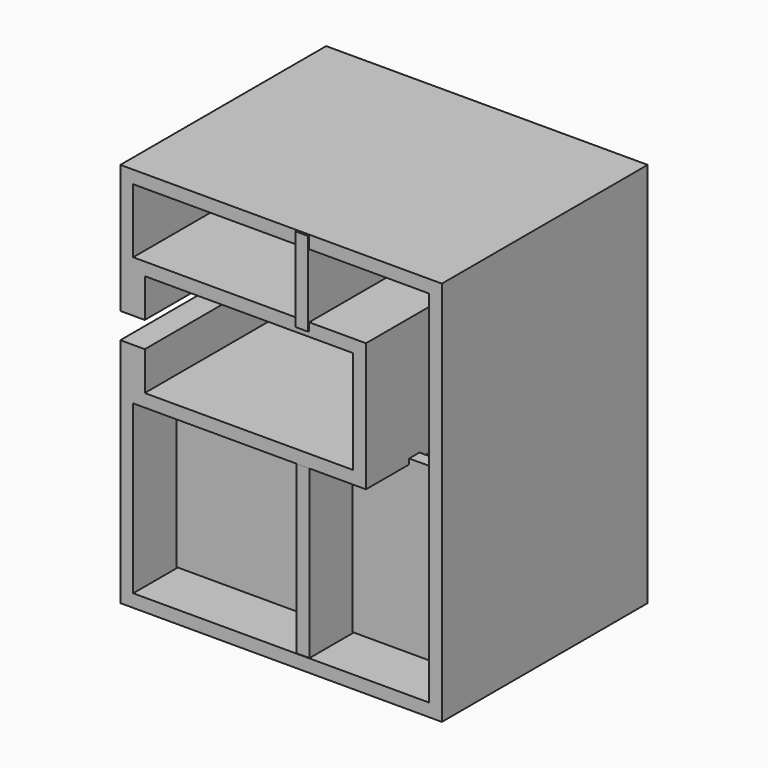
from build123d import *

# Parameters (mm, degrees)
F0_W         = 63.5
F0_H         = 50.8
F1_DEPTH     = 76.2
F3_DEPTH     = 38.1
F4_T         = 2.54
F4_T3_DEPTH  = 9.906
F4_T5_DEPTH  = 46.228
F4_T7_DEPTH  = 12.7
F4_T9_DEPTH  = 12.7
F4_T11_DEPTH = 25.4
F4_T13_DEPTH = 43.18
F5_W         = 49.4960099459
F5_H         = 36.6942100227
F5_W_2       = 49.6212309226
F5_H_2       = 16.634516418
F6_DEPTH     = 1.27
F7_W         = 57.8342098743
F7_H         = 36.6147905588
F8_DEPTH     = 1.27
F10_W        = 61.5059640259
F10_H        = 33.8196810335
F11_DEPTH    = 1.27


# Not quite as in the source:
# - a shell that OpenCascade refuses in one call is made with other operations: the cavity is built on its own and cut out


with BuildPart() as f1:
    # F0 (on Top) → F1 (new body)
    with BuildSketch(Plane.XY):
        with Locations((-4.2696721688, -14.4747652373)):
            Rectangle(F0_W, F0_H)
    extrude(amount=F1_DEPTH)

    # F2 (on face) → F3 (cut)
    with BuildSketch(Plane.XZ.offset(39.8747652373)):
        Polygon((9.9543278312, 58.42), (-31.1936721688, 58.42), (-31.1936721688, 50.8), (-39.8653410375, 50.8), (-39.8653410375, 45.72), (-31.1936721688, 45.72), (-31.1936721688, 38.1), (9.9543278312, 38.1), align=None)
    extrude(amount=-F3_DEPTH, mode=Mode.SUBTRACT)

    # F4: shell of thickness 2.54, made by hand


with BuildPart() as f4_core1:
    # F4_t2: copy of F1
    add(f1.part)

    # the walls: a layer under each face that stays
    f4_faces = [f4_core1.faces().sort_by_distance(p)[0] for p in [
        (-4.2696721688, 10.9252347627, 38.1),
        (27.4803278312, -14.4747652373, 38.1),
        (-36.0196721688, -14.4747652373, 38.1),
        (-4.2696721688, -14.4747652373, 0),
        (-4.2696721688, -14.4747652373, 76.2),
        (-33.6066721688, -20.8247652373, 45.72),
        (-13.0326721688, -1.7747652373, 48.26),
        (-33.6066721688, -20.8247652373, 50.8),
        (-31.1936721688, -20.8247652373, 54.61),
        (-10.6196721688, -20.8247652373, 58.42),
        (9.9543278312, -20.8247652373, 48.26),
        (-10.6196721688, -20.8247652373, 38.1),
        (-31.1936721688, -20.8247652373, 41.91),
    ]]
    thicken(f4_faces, amount=-F4_T, mode=Mode.SUBTRACT)

    # F4_s4 → F4_t3 (cut)
    with BuildSketch(Plane.YZ.offset(-38.5596721688)):
        Polygon((-1.8001652373, 45.7454), (-1.7747652373, 43.18), (0.7652347627, 43.18), (0.7652347627, 45.72), align=None)
        Polygon((-1.8001652373, 50.7746), (0.7652347627, 50.8), (0.7652347627, 53.34), (-1.7747652373, 53.34), align=None)
    extrude(amount=F4_T3_DEPTH, mode=Mode.SUBTRACT)

    # F4_s6 → F4_t5 (cut)
    with BuildSketch(Plane.YZ.offset(-33.7336721688)):
        Polygon((-1.8001652373, 38.1254), (0.7652347627, 38.1), (0.7652347627, 35.56), (-1.7747652373, 35.56), align=None)
        Polygon((-1.8001652373, 58.3946), (0.7652347627, 58.42), (0.7652347627, 60.96), (-1.7747652373, 60.96), align=None)
    extrude(amount=F4_T5_DEPTH, mode=Mode.SUBTRACT)

    # F4_s8 → F4_t7 (cut)
    with BuildSketch(Plane.XY.offset(35.56)):
        Polygon((-31.1682721688, -1.8001652373), (-31.1936721688, 0.7652347627), (-33.7336721688, 0.7652347627), (-33.7336721688, -1.7747652373), align=None)
    extrude(amount=F4_T7_DEPTH, mode=Mode.SUBTRACT)

    # F4_s10 → F4_t9 (cut)
    with BuildSketch(Plane.XY.offset(48.26)):
        Polygon((-31.1682721688, -1.8001652373), (-31.1936721688, 0.7652347627), (-33.7336721688, 0.7652347627), (-33.7336721688, -1.7747652373), align=None)
    extrude(amount=F4_T9_DEPTH, mode=Mode.SUBTRACT)

    # F4_s12 → F4_t11 (cut)
    with BuildSketch(Plane.XY.offset(35.56)):
        Polygon((9.9289278312, -1.8001652373), (9.9543278312, 0.7652347627), (12.4943278312, 0.7652347627), (12.4943278312, -1.7747652373), align=None)
    extrude(amount=F4_T11_DEPTH, mode=Mode.SUBTRACT)

    # F4_s14 → F4_t13 (cut)
    with BuildSketch(Plane.XZ.offset(-0.7652347627)):
        Polygon((-31.1682721688, 58.3946), (-33.7336721688, 58.42), (-33.7336721688, 60.96), (-31.1936721688, 60.96), align=None)
        Polygon((9.9289278312, 58.3946), (9.9543278312, 60.96), (12.4943278312, 60.96), (12.4943278312, 58.42), align=None)
        Polygon((9.9289278312, 38.1254), (12.4943278312, 38.1), (12.4943278312, 35.56), (9.9543278312, 35.56), align=None)
        Polygon((-31.1682721688, 38.1254), (-31.1936721688, 35.56), (-33.7336721688, 35.56), (-33.7336721688, 38.1), align=None)
    extrude(amount=F4_T13_DEPTH, mode=Mode.SUBTRACT)


with BuildPart() as f1_1:
    add(f1.part)

    # what is left inside the walls is the cavity
    f4_cavity = [f4_core1.part.solids().sort_by_distance(p)[0] for p in [
        (-4.269672, 8.359835, 49.953333),
    ]]
    add(f4_cavity, mode=Mode.SUBTRACT)

    # F5 (on Right) → F6 (join, symmetric)
    with BuildSketch(Plane.YZ):
        with Locations((-15.0325410068, 18.3471050113)):
            Rectangle(F5_W, F5_H)
        with Locations((-15.3072369285, 67.7350275218)):
            Rectangle(F5_W_2, F5_H_2)
    extrude(amount=F6_DEPTH, both=True)

    # F7 (on Front) → F8 (join, symmetric)
    with BuildSketch(Plane.XZ):
        with Locations((-4.0594032034, 18.3073952794)):
            Rectangle(F7_W, F7_H)
    extrude(amount=F8_DEPTH, both=True)

    # F10 (on offset) → F11 (join, symmetric)
    with BuildSketch(Plane.XZ.offset(27.94)):
        with Locations((-4.893549718, 19.6837866679)):
            Rectangle(F10_W, F10_H)
    extrude(amount=F11_DEPTH, both=True)


solid = f1_1.part
